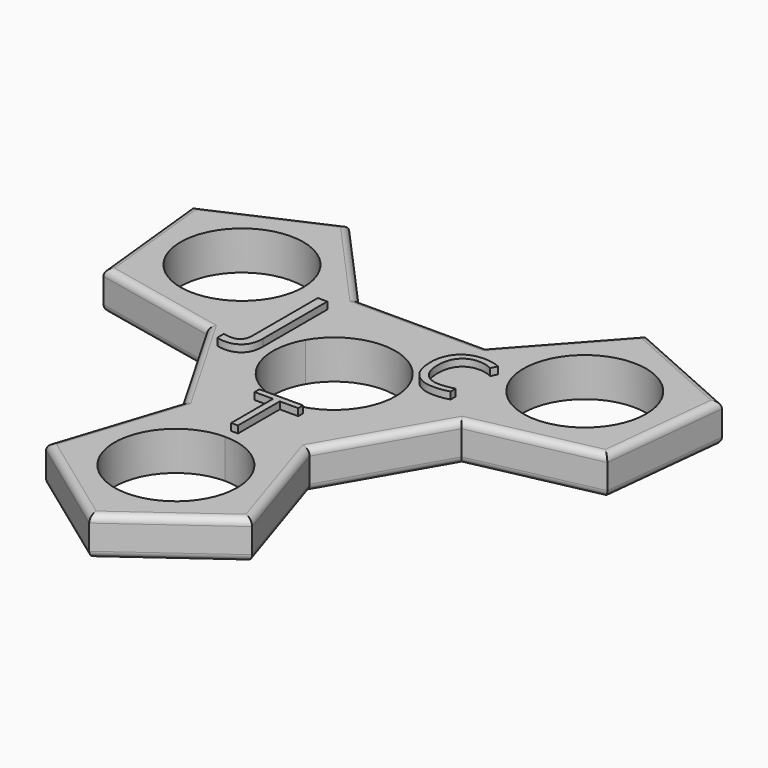
from build123d import *

# Parameters (mm, degrees)
F1_DEPTH       = 6.985
F2_TEXT_SIZE   = 20.4407510146
F2_TEXT_SIZE_2 = 15.1490843479
F2_TEXT_SIZE_3 = 14.6506751132
F3_DEPTH       = 1.27
F4_R           = 1.27


# Not quite as in the source:
# - Text() gives the source's letters only with a copy of the font that has no kerning and outlines rounded to 1/6400 em; it was checked with that copy


with BuildPart() as f1:
    # F0 (on Top) → F1 (new body)
    with BuildSketch(Plane.XY):
        with BuildLine():
            ThreePointArc((9.5357191185, 5.50545), (10.6357126807, 2.8498306237), (11.0109, 0))
            ThreePointArc((11.0109, 0), (7.785882057, -7.785882057), (0, -11.0109))
            Line((0, -11.0109), (0, -19.7973407305))
            Line((0, -19.7973407305), (11.43, -19.7973407305))
            Line((11.43, -19.7973407305), (22.86, 0))
            Line((22.86, 0), (17.145, 9.8986703653))
            Line((17.145, 9.8986703653), (9.5357191185, 5.50545))
        make_face()
        with BuildLine():
            ThreePointArc((-9.5357191185, 5.50545), (0, 11.0109), (9.5357191185, 5.50545))
            Line((9.5357191185, 5.50545), (17.145, 9.8986703653))
            Line((17.145, 9.8986703653), (11.43, 19.7973407305))
            Line((11.43, 19.7973407305), (-11.43, 19.7973407305))
            Line((-11.43, 19.7973407305), (-17.145, 9.8986703653))
            Line((-17.145, 9.8986703653), (-9.5357191185, 5.50545))
        make_face()
        with BuildLine():
            Line((0, -19.7973407305), (0, -11.0109))
            ThreePointArc((0, -11.0109), (-9.5357191185, -5.50545), (-9.5357191185, 5.50545))
            Line((-9.5357191185, 5.50545), (-17.145, 9.8986703653))
            Line((-17.145, 9.8986703653), (-22.86, 0))
            Line((-22.86, 0), (-11.43, -19.7973407305))
            Line((-11.43, -19.7973407305), (0, -19.7973407305))
        make_face()
        Polygon((11.43, 19.7973407305), (17.145, 9.8986703653), (22.86, 0), (45.2204541528, 4.7528612521), (47.6099748231, 27.4876317802), (26.7263256614, 36.7856314409), align=None)
        with BuildLine():
            ThreePointArc((41.7802509274, 17.7646930407), (33.6191815512, 7.1289803601), (21.2336318089, 12.2592430407))
            ThreePointArc((21.2336318089, 12.2592430407), (27.9195203037, 28.4004057214), (41.7802509274, 17.7646930407))
        make_face(mode=Mode.SUBTRACT)
        Polygon((11.43, -19.7973407305), (0, -19.7973407305), (-11.43, -19.7973407305), (-18.4941284914, -41.538492693), (0, -54.9752635604), (18.4941284914, -41.538492693), align=None)
        with BuildLine():
            ThreePointArc((11.0109, -35.5293860815), (-7.785882057, -43.3152681385), (0, -24.5184860815))
            ThreePointArc((0, -24.5184860815), (7.785882057, -27.7435040245), (11.0109, -35.5293860815))
        make_face(mode=Mode.SUBTRACT)
        Polygon((-22.86, 0), (-17.145, 9.8986703653), (-11.43, 19.7973407305), (-26.7263256614, 36.7856314409), (-47.6099748231, 27.4876317802), (-45.2204541528, 4.7528612521), align=None)
        with BuildLine():
            ThreePointArc((-19.7584509274, 17.7646930407), (-20.1336382468, 14.914862417), (-21.2336318089, 12.2592430407))
            ThreePointArc((-21.2336318089, 12.2592430407), (-41.4050636081, 20.6145236645), (-19.7584509274, 17.7646930407))
        make_face(mode=Mode.SUBTRACT)
    extrude(amount=F1_DEPTH)

    # F2 (on face) → F3 (join)
    with BuildSketch(Plane.XY.offset(6.985)):
        with Locations((-16.51, 0)):
            Text('J', F2_TEXT_SIZE, font='Open Sans', text_align=(TextAlign.LEFT, TextAlign.BOTTOM))
        with Locations((8.961656642, 3.81)):
            Text('C', F2_TEXT_SIZE_2, font='Open Sans', text_align=(TextAlign.LEFT, TextAlign.BOTTOM))
        with Locations((-3.8385984752, -22.6134860815)):
            Text('T', F2_TEXT_SIZE_3, font='Open Sans', text_align=(TextAlign.LEFT, TextAlign.BOTTOM))
    extrude(amount=F3_DEPTH)

    # F4
    f4_edges = [f1.edges().sort_by_distance(p)[0] for p in [
        (0, 19.797341, 6.985),
        (19.078163, 28.291486, 6.985),
        (14.962064, -30.667917, 6.985),
        (9.247064, -48.256878, 6.985),
        (-9.247064, -48.256878, 6.985),
        (-14.962064, -30.667917, 6.985),
        (17.145, -9.89867, 6.985),
        (34.040227, 2.376431, 6.985),
        (46.415214, 16.120247, 6.985),
        (37.16815, 32.136632, 6.985),
        (-19.078163, 28.291486, 6.985),
        (-37.16815, 32.136632, 6.985),
        (-46.415214, 16.120247, 6.985),
        (-34.040227, 2.376431, 6.985),
        (-17.145, -9.89867, 6.985),
        (0, 19.797341, 0),
        (-19.078163, 28.291486, 0),
        (-37.16815, 32.136632, 0),
        (-46.415214, 16.120247, 0),
        (-34.040227, 2.376431, 0),
        (-17.145, -9.89867, 0),
        (-14.962064, -30.667917, 0),
        (-9.247064, -48.256878, 0),
        (9.247064, -48.256878, 0),
        (14.962064, -30.667917, 0),
        (17.145, -9.89867, 0),
        (34.040227, 2.376431, 0),
        (46.415214, 16.120247, 0),
        (37.16815, 32.136632, 0),
        (19.078163, 28.291486, 0),
    ]]
    fillet(f4_edges, radius=F4_R)


solid = f1.part
